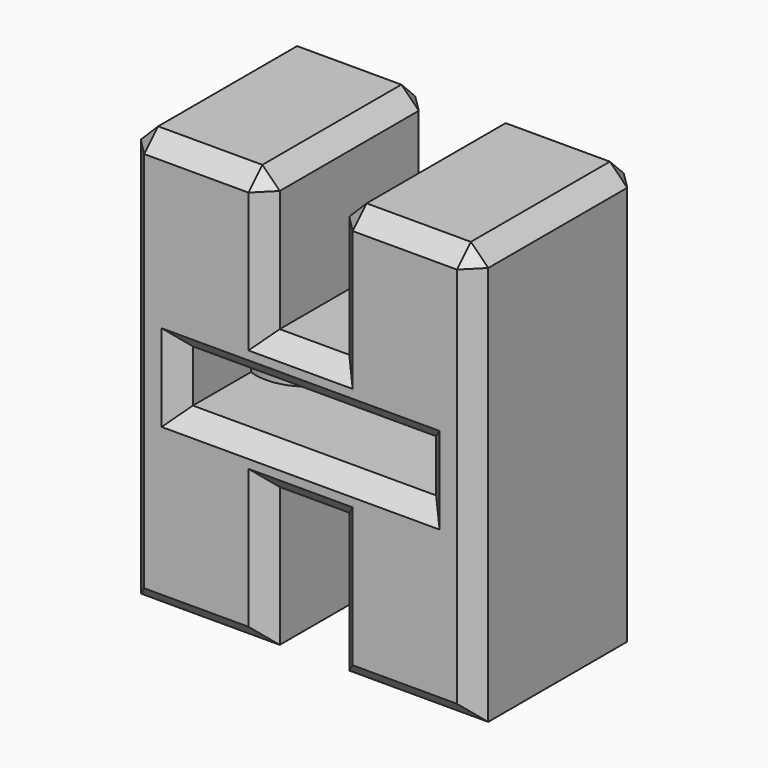
from build123d import *

# Parameters (mm, degrees)
F1_DEPTH = 60
F2_W     = 70
F2_H     = 15
F3_DEPTH = 50
F4_R     = 15
F5_R     = 15
F6_DEPTH = 67.5
F7_SIZE  = 5
F8_SIZE  = 4.99999
F9_SIZE  = 5


# Not quite as in the source:
# - a fillet or chamfer is up to 0.001 mm smaller than in the source, because OpenCascade refuses the exact size


with BuildPart() as f1:
    # F0 (on Front) → F1 (new body)
    with BuildSketch(Plane.XZ):
        Polygon((-8.0390890029, 59.2476050396), (-48.0390890029, 59.2476050396), (-48.0390890029, -60.7523949604), (-8.0390890029, -60.7523949604), (-8.0390890029, -20.7523949604), (11.9609109971, -20.7523949604), (11.9609109971, -60.7523949604), (51.9609109971, -60.7523949604), (51.9609109971, 59.2476050396), (11.9609109971, 59.2476050396), (11.9609109971, 19.2476050396), (-8.0390890029, 19.2476050396), align=None)
    extrude(amount=F1_DEPTH)

    # F2 (on face) → F3 (cut)
    with BuildSketch(Plane.XZ.offset(60)):
        with Locations((1.9609109971, -0.7523949604)):
            Rectangle(F2_W, F2_H)
    extrude(amount=-F3_DEPTH, mode=Mode.SUBTRACT)

    # F4 (on face) + F5 (on face) → F6 (cut)
    with BuildSketch(Plane(origin=(0, 0, -60.7523949604), x_dir=(1, 0, 0), z_dir=(0, 0, -1))):
        with Locations((-28.0390890029, 20)):
            Circle(F4_R)
    with BuildSketch(Plane(origin=(0, 0, -60.7523949604), x_dir=(1, 0, 0), z_dir=(0, 0, -1))):
        with Locations((31.9609109971, 20)):
            Circle(F5_R)
    extrude(amount=-F6_DEPTH, mode=Mode.SUBTRACT)

    # F7
    f7_edges = [f1.edges().sort_by_distance(p)[0] for p in [
        (-48.039089, -30, 59.247605),
        (-8.039089, -30, 59.247605),
        (11.960911, -30, 59.247605),
        (51.960911, -30, 59.247605),
        (31.960911, -60, 59.247605),
        (-28.039089, -60, 59.247605),
        (31.960911, 0, 59.247605),
        (-28.039089, 0, 59.247605),
        (1.960911, -60, 6.747605),
        (-33.039089, -60, -0.752395),
        (1.960911, -60, -8.252395),
        (36.960911, -60, -0.752395),
        (51.960911, -60, -0.752395),
        (51.960911, 0, -0.752395),
        (11.960911, -60, 39.247605),
        (1.960911, -60, 19.247605),
        (-8.039089, -60, 39.247605),
        (31.960911, -60, -60.752395),
        (11.960911, -60, -40.752395),
        (-48.039089, -60, -0.752395),
        (1.960911, -60, -20.752395),
        (-28.039089, -60, -60.752395),
        (-8.039089, -60, -40.752395),
        (-48.039089, 0, -0.752395),
        (11.960911, 0, -40.752395),
        (-8.039089, 0, -40.752395),
        (11.960911, 0, 39.247605),
        (-8.039089, 0, 39.247605),
    ]]
    chamfer(f7_edges, length=F7_SIZE)

    # F8 (size 5 in the source; OpenCascade refuses exactly that, so slightly less here)
    f8_edges = [f1.edges().sort_by_distance(p)[0] for p in [
        (1.960911, 0, -20.752395),
    ]]
    chamfer(f8_edges, length=F8_SIZE)

    # F9
    f9_edges = [f1.edges().sort_by_distance(p)[0] for p in [
        (1.960911, 0, 19.247605),
    ]]
    chamfer(f9_edges, length=F9_SIZE)


solid = f1.part
